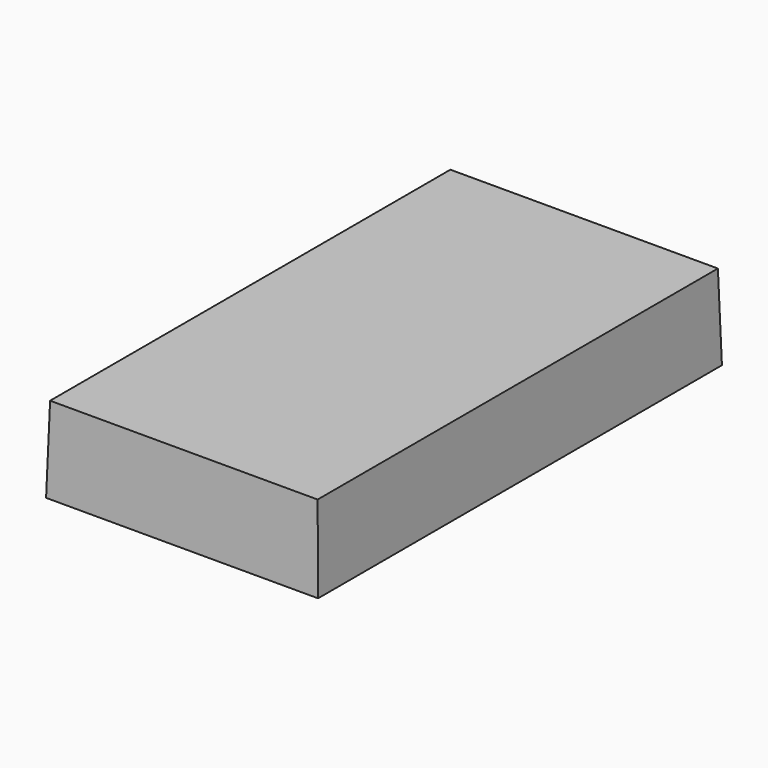
from build123d import *

# Parameters (mm, degrees)
F0_W          = 35.2
F0_H          = 68.2
F1_DEPTH      = 10
F2_W          = 6.5
F2_H          = 14
F3_DEPTH      = 1
F5_W          = 42
F5_H          = 78
F6_DEPTH      = 12
F6_TAPER      = 1.5
F6_DEPTH_BACK = 1.2
F6_TAPER_BACK = -1.5
F7_T          = -1.8
F8_W          = 38.2616121588
F8_H          = 74.2616121588
F9_DEPTH      = 1.2
F10_W         = 15
F10_H         = 1.2
F11_DEPTH     = 10
F13_DEPTH     = 15


with BuildPart() as f1:
    # F0 (on Top) → F1 (new body)
    with BuildSketch(Plane.XY):
        Rectangle(F0_W, F0_H)
    extrude(amount=F1_DEPTH)

    # F2 (on face) → F3 (cut)
    with BuildSketch(Plane.XY.offset(10)):
        with Locations((13.35, -26)):
            Rectangle(F2_W, F2_H)
    extrude(amount=-F3_DEPTH, mode=Mode.SUBTRACT)


with BuildPart() as f6:
    # F5 (on face) → F6 (new body, two sides)
    with BuildSketch(Plane(origin=(0, 0, 0), x_dir=(1, 0, 0), z_dir=(0, 0, -1))) as f6_sk:
        Rectangle(F5_W, F5_H)
    extrude(amount=-F6_DEPTH, taper=F6_TAPER)
    extrude(f6_sk.sketch, amount=F6_DEPTH_BACK, taper=F6_TAPER_BACK)

    # F7
    f7_openings = [f6.faces().sort_by_distance(p)[0] for p in [
        (0, 0, -1.2),
    ]]
    offset(amount=F7_T, openings=f7_openings)


with BuildPart() as f9:
    # F8 (on face) → F9 (new body)
    with BuildSketch(Plane(origin=(0, 0, 0), x_dir=(1, 0, 0), z_dir=(0, 0, -1))):
        Rectangle(F8_W, F8_H)
    extrude(amount=F9_DEPTH)

    # F10 (on face) → F11 (join)
    with BuildSketch(Plane.XY):
        with Locations((0, -36.5308060794)):
            Rectangle(F10_W, F10_H)
    extrude(amount=F11_DEPTH)

    # F12 (on face) → F13 (join, through all)
    with BuildSketch(Plane(origin=(-7.5, 0, 0), x_dir=(0, -1, 0), z_dir=(-1, 0, 0))):
        Polygon((37.1308060794, 7), (37.1308060794, 5.4), (37.9308060794, 5.4), align=None)
    extrude(amount=-F13_DEPTH)


solid = Compound([f1.part, f6.part, f9.part])
